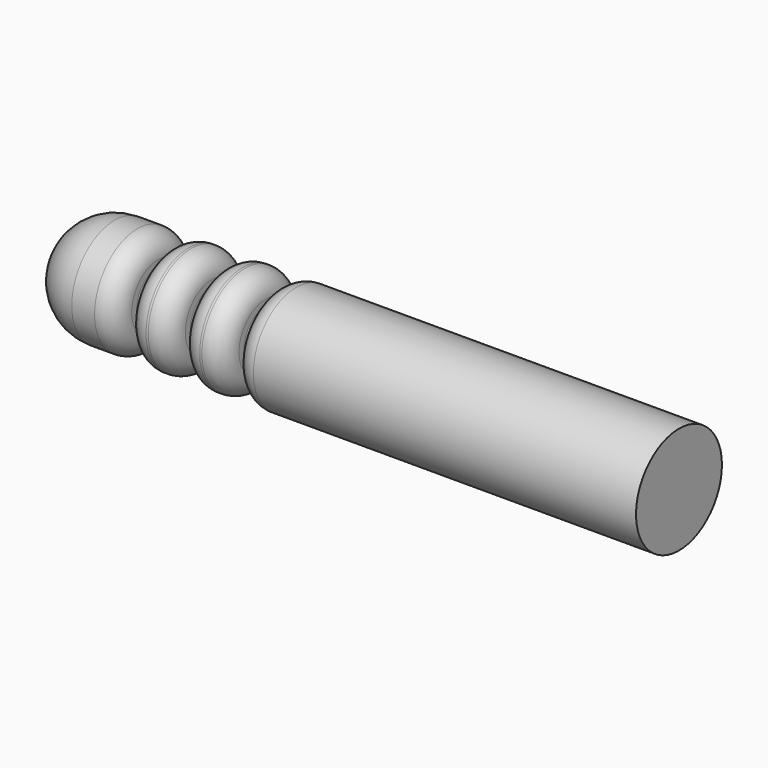
from build123d import *

# Parameters (mm, degrees)
F2_R = 5.08
F3_R = 1.26999


# Not quite as in the source:
# - a fillet or chamfer is up to 0.001 mm smaller than in the source, because OpenCascade refuses the exact size


with BuildPart() as f1:
    # F0 (on Top) → F1 (revolve)
    with BuildSketch(Plane.XY):
        with BuildLine():
            Line((-52.0266967201, 13.2484138012), (-62.7351105213, 13.2484138012))
            ThreePointArc((-62.7351105213, 13.2484138012), (-72.1031537601, 9.3680432388), (-75.9835243225, 0))
            Line((-75.9835243225, 0), (76.5030682087, 0))
            Line((76.5030682087, 0), (76.5030682087, 13.2484138012))
            Line((76.5030682087, 13.2484138012), (-22.9898691177, 13.2484138012))
            Line((-22.9898691177, 13.2484138012), (-22.9898691177, 5.3568566218))
            Line((-22.9898691177, 5.3568566218), (-25.5298691177, 5.3568566218))
            Line((-25.5298691177, 5.3568566218), (-25.5298691177, 13.2484138012))
            Line((-25.5298691177, 13.2484138012), (-36.2382829189, 13.2484138012))
            Line((-36.2382829189, 13.2484138012), (-36.2382829189, 5.3568566218))
            Line((-36.2382829189, 5.3568566218), (-38.7782829189, 5.3568566218))
            Line((-38.7782829189, 5.3568566218), (-38.7782829189, 13.2484138012))
            Line((-38.7782829189, 13.2484138012), (-49.4866967201, 13.2484138012))
            Line((-49.4866967201, 13.2484138012), (-49.4866967201, 5.3568566218))
            Line((-49.4866967201, 5.3568566218), (-52.0266967201, 5.3568566218))
            Line((-52.0266967201, 5.3568566218), (-52.0266967201, 13.2484138012))
        make_face()
    revolve(axis=Axis((0.2597719431, 0, 0), (-1, 0, 0)))

    # F2
    f2_edges = [f1.edges().sort_by_distance(p)[0] for p in [
        (-52.026697, -13.248414, 0),
        (-49.486697, -13.248414, 0),
        (-38.778283, -13.248414, 0),
        (-36.238283, -13.248414, 0),
        (-25.529869, -13.248414, 0),
        (-22.989869, -13.248414, 0),
    ]]
    fillet(f2_edges, radius=F2_R)

    # F3 (radius 1.27 in the source; OpenCascade refuses exactly that, so slightly less here)
    f3_edges = [f1.edges().sort_by_distance(p)[0] for p in [
        (-49.486697, -5.356857, 0),
        (-52.026697, -5.356857, 0),
        (-36.238283, -5.356857, 0),
        (-38.778283, -5.356857, 0),
        (-25.529869, -5.356857, 0),
        (-22.989869, -5.356857, 0),
    ]]
    fillet(f3_edges, radius=F3_R)


solid = f1.part
